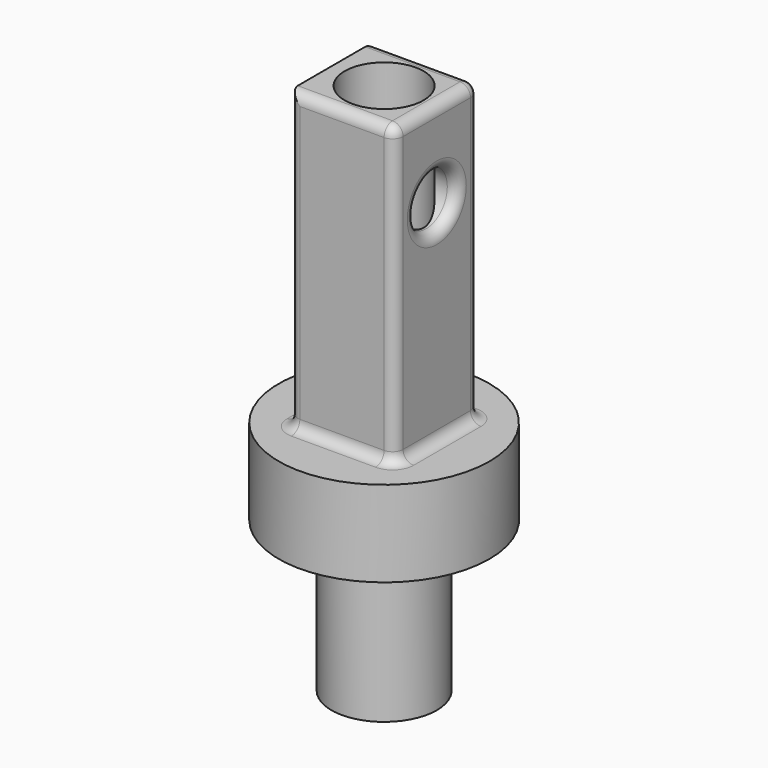
from build123d import *

# Parameters (mm, degrees)
F0_R      = 50.8
F1_DEPTH  = 41.4476916194
F2_W      = 50.8
F2_H      = 50.8
F3_DEPTH  = 143.017962575
F4_R      = 12.7
F5_DEPTH  = 76.201
F6_R      = 5.08
F7_R      = 19.05
F8_DEPTH  = 184.4666541944
F9_R      = 25.4
F9_R_2    = 19.05
F10_DEPTH = 72.4607035518


with BuildPart() as f1:
    # F0 (on Top) → F1 (new body)
    with BuildSketch(Plane.XY):
        Circle(F0_R)
    extrude(amount=-F1_DEPTH)

    # F2 (on face) → F3 (join)
    with BuildSketch(Plane.XY):
        Rectangle(F2_W, F2_H)
    extrude(amount=F3_DEPTH)

    # F4 (on face) → F5 (cut, through all)
    with BuildSketch(Plane.YZ.offset(25.4)):
        with Locations((0, 101.6)):
            Circle(F4_R)
    extrude(amount=-F5_DEPTH, mode=Mode.SUBTRACT)

    # F6
    f6_edges = [f1.edges().sort_by_distance(p)[0] for p in [
        (25.4, 25.4, 71.508981),
        (-25.4, 25.4, 71.508981),
        (0, 25.4, 0),
        (0, 25.4, 143.017963),
        (25.4, -25.4, 71.508981),
        (25.4, 0, 0),
        (25.4, 0, 143.017963),
        (25.4, -12.7, 101.6),
        (-25.4, -25.4, 71.508981),
        (0, -25.4, 0),
        (0, -25.4, 143.017963),
        (-25.4, 0, 0),
    ]]
    fillet(f6_edges, radius=F6_R)

    # F7 (on face) → F8 (cut, through all)
    with BuildSketch(Plane(origin=(0, 0, -41.4476916194), x_dir=(1, 0, 0), z_dir=(0, 0, -1))):
        Circle(F7_R)
    extrude(amount=-F8_DEPTH, mode=Mode.SUBTRACT)

    # F9 (on face) → F10 (join)
    with BuildSketch(Plane(origin=(0, 0, -41.4476916194), x_dir=(1, 0, 0), z_dir=(0, 0, -1))):
        Circle(F9_R)
        Circle(F9_R_2, mode=Mode.SUBTRACT)
    extrude(amount=F10_DEPTH)


solid = f1.part
